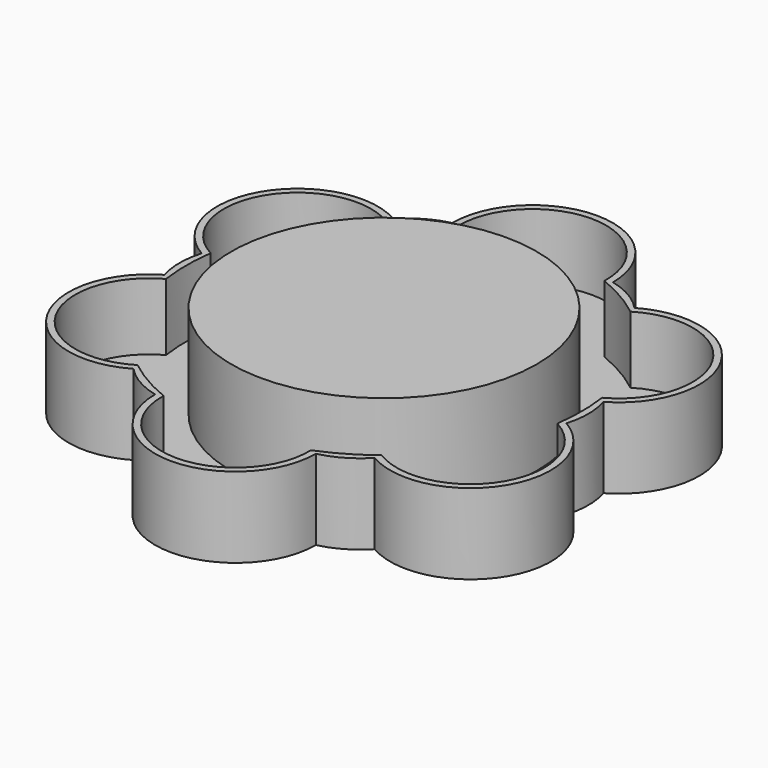
from build123d import *

# Parameters (mm, degrees)
F0_R        = 72.39
F1_DEPTH    = 6.35
F2_DEPTH    = 50.8
F3_T1_DEPTH = 69.85
F5_DEPTH    = 31.75


# Not quite as in the source:
# - a fillet or chamfer that OpenCascade refuses, or shapes differently, is made with other operations: its cross-section is extruded or revolved along the edge and cut away or added


with BuildPart() as f1:
    # F0 (on Top) → F1 (new body)
    with BuildSketch(Plane.XY):
        with BuildLine():
            Line((38.1, -87.9881810245), (50.8, -87.9881810245))
            Line((50.8, -87.9881810245), (57.15, -76.9896583964))
            ThreePointArc((57.15, -76.9896583964), (109.1955678842, -63.0440905122), (95.25, -10.9985226281))
            Line((95.25, -10.9985226281), (101.6, 0))
            Line((101.6, 0), (95.25, 10.9985226281))
            ThreePointArc((95.25, 10.9985226281), (109.1955678842, 63.0440905122), (57.15, 76.9896583964))
            Line((57.15, 76.9896583964), (50.8, 87.9881810245))
            Line((50.8, 87.9881810245), (38.1, 87.9881810245))
            ThreePointArc((38.1, 87.9881810245), (0, 126.0881810245), (-38.1, 87.9881810245))
            Line((-38.1, 87.9881810245), (-50.8, 87.9881810245))
            Line((-50.8, 87.9881810245), (-57.15, 76.9896583964))
            ThreePointArc((-57.15, 76.9896583964), (-109.1955678842, 63.0440905122), (-95.25, 10.9985226281))
            Line((-95.25, 10.9985226281), (-101.6, 0))
            Line((-101.6, 0), (-95.25, -10.9985226281))
            ThreePointArc((-95.25, -10.9985226281), (-109.1955678842, -63.0440905122), (-57.15, -76.9896583964))
            Line((-57.15, -76.9896583964), (-50.8, -87.9881810245))
            Line((-50.8, -87.9881810245), (-38.1, -87.9881810245))
            ThreePointArc((-38.1, -87.9881810245), (0, -126.0881810245), (38.1, -87.9881810245))
        make_face()
        Circle(F0_R, mode=Mode.SUBTRACT)
    extrude(amount=F1_DEPTH)

    # F0 (on Top) → F2 (join)
    with BuildSketch(Plane.XY):
        Circle(F0_R)
    extrude(amount=F2_DEPTH)

    # F3: fillet of radius 38.1 on 6 edges, made by hand

    # F3_s2 → F3_t1 (cut)
    with BuildSketch(Plane.XY.offset(-31.75)):
        with BuildLine():
            ThreePointArc((57.15, 76.9896583964), (48.4360135972, 83.8936364665), (38.1, 87.9881810245))
            Line((38.1, 87.9881810245), (50.8, 87.9881810245))
            Line((50.8, 87.9881810245), (57.15, 76.9896583964))
        make_face()
        with BuildLine():
            ThreePointArc((95.25, -10.9985226281), (96.8720271945, 0), (95.25, 10.9985226281))
            Line((95.25, 10.9985226281), (101.6, 0))
            Line((101.6, 0), (95.25, -10.9985226281))
        make_face()
        with BuildLine():
            ThreePointArc((38.1, -87.9881810245), (48.4360135972, -83.8936364665), (57.15, -76.9896583964))
            Line((57.15, -76.9896583964), (50.8, -87.9881810245))
            Line((50.8, -87.9881810245), (38.1, -87.9881810245))
        make_face()
        with BuildLine():
            ThreePointArc((-38.1, -87.9881810245), (-48.4360135972, -83.8936364665), (-57.15, -76.9896583964))
            Line((-57.15, -76.9896583964), (-50.8, -87.9881810245))
            Line((-50.8, -87.9881810245), (-38.1, -87.9881810245))
        make_face()
        with BuildLine():
            ThreePointArc((-95.25, 10.9985226281), (-96.8720271945, 0), (-95.25, -10.9985226281))
            Line((-95.25, -10.9985226281), (-101.6, 0))
            Line((-101.6, 0), (-95.25, 10.9985226281))
        make_face()
        with BuildLine():
            ThreePointArc((-38.1, 87.9881810245), (-48.4360135972, 83.8936364665), (-57.15, 76.9896583964))
            Line((-57.15, 76.9896583964), (-50.8, 87.9881810245))
            Line((-50.8, 87.9881810245), (-38.1, 87.9881810245))
        make_face()
    extrude(amount=F3_T1_DEPTH, mode=Mode.SUBTRACT)

    # F4 (on face) → F5 (join)
    with BuildSketch(Plane.XY.offset(6.35)):
        with BuildLine():
            ThreePointArc((-95.25, -10.9985226281), (-109.1955678842, -63.0440905122), (-57.15, -76.9896583964))
            ThreePointArc((-57.15, -76.9896583964), (-48.4360135972, -83.8936364665), (-38.1, -87.9881810245))
            ThreePointArc((-38.1, -87.9881810245), (0, -126.0881810245), (38.1, -87.9881810245))
            ThreePointArc((38.1, -87.9881810245), (48.4360135972, -83.8936364665), (57.15, -76.9896583964))
            ThreePointArc((57.15, -76.9896583964), (109.1955678842, -63.0440905122), (95.25, -10.9985226281))
            ThreePointArc((95.25, -10.9985226281), (96.8720271945, 0), (95.25, 10.9985226281))
            ThreePointArc((95.25, 10.9985226281), (109.1955678842, 63.0440905122), (57.15, 76.9896583964))
            ThreePointArc((57.15, 76.9896583964), (48.4360135972, 83.8936364665), (38.1, 87.9881810245))
            ThreePointArc((38.1, 87.9881810245), (0, 126.0881810245), (-38.1, 87.9881810245))
            ThreePointArc((-38.1, 87.9881810245), (-48.4360135972, 83.8936364665), (-57.15, 76.9896583964))
            ThreePointArc((-57.15, 76.9896583964), (-109.1955678842, 63.0440905122), (-95.25, 10.9985226281))
            ThreePointArc((-95.25, 10.9985226281), (-96.8720271945, 0), (-95.25, -10.9985226281))
        make_face()
        with BuildLine():
            ThreePointArc((-92.7564557809, 13.2428401804), (-106.4459372272, 61.4565905122), (-57.8468639049, 73.7080269811))
            ThreePointArc((-57.8468639049, 73.7080269811), (-46.8485135972, 81.1440058095), (-34.909591876, 86.9508671615))
            ThreePointArc((-34.909591876, 86.9508671615), (0, 122.9131810245), (34.909591876, 86.9508671615))
            ThreePointArc((34.909591876, 86.9508671615), (46.8485135972, 81.1440058095), (57.8468639049, 73.7080269811))
            ThreePointArc((57.8468639049, 73.7080269811), (106.4459372272, 61.4565905122), (92.7564557809, 13.2428401804))
            ThreePointArc((92.7564557809, 13.2428401804), (93.6970271945, 0), (92.7564557809, -13.2428401804))
            ThreePointArc((92.7564557809, -13.2428401804), (106.4459372272, -61.4565905122), (57.8468639049, -73.7080269811))
            ThreePointArc((57.8468639049, -73.7080269811), (46.8485135972, -81.1440058095), (34.909591876, -86.9508671615))
            ThreePointArc((34.909591876, -86.9508671615), (0, -122.9131810245), (-34.909591876, -86.9508671615))
            ThreePointArc((-34.909591876, -86.9508671615), (-46.8485135972, -81.1440058095), (-57.8468639049, -73.7080269811))
            ThreePointArc((-57.8468639049, -73.7080269811), (-106.4459372272, -61.4565905122), (-92.7564557809, -13.2428401804))
            ThreePointArc((-92.7564557809, -13.2428401804), (-93.6970271945, 0), (-92.7564557809, 13.2428401804))
        make_face(mode=Mode.SUBTRACT)
    extrude(amount=F5_DEPTH)


solid = f1.part
